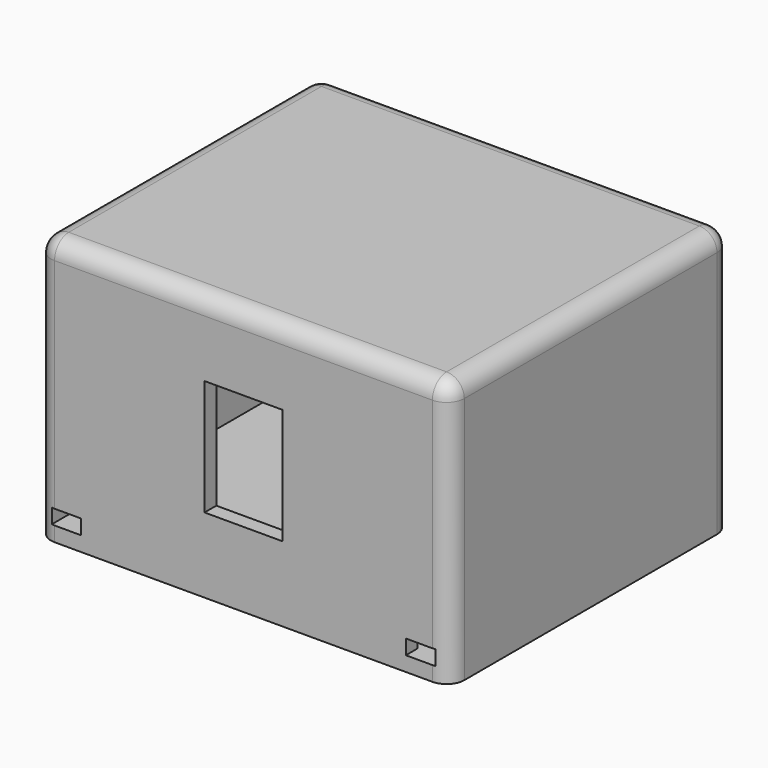
from build123d import *

# Parameters (mm, degrees)
F0_W         = 70
F0_H         = 45
F0_W_2       = 20.7
F0_H_2       = 27.2
F0_W_3       = 25.5
F0_H_3       = 32.8
F1_DEPTH     = 2
F2_W         = 70
F2_H         = 45
F2_W_2       = 65
F2_H_2       = 40
F3_DEPTH     = 55
F4_W         = 70
F4_H         = 45
F4_W_2       = 13.2
F4_H_2       = 19.6
F5_DEPTH     = 2.5
F6_W         = 5
F6_H         = 2.5
F7_DEPTH     = 59.501
F8_T1_DEPTH  = 64
F8_T3_DEPTH  = 49.5
F8_T5_DEPTH  = 53.5
F8_S9_W      = 3
F8_S9_H      = 3
F8_T10_DEPTH = 3
F8_S15_W     = 3
F8_S15_H     = 3
F8_T16_DEPTH = 3
F8_S21_W     = 3
F8_S21_H     = 3
F8_T22_DEPTH = 3
F8_S27_W     = 3
F8_S27_H     = 3
F8_T28_DEPTH = 3


# Not quite as in the source:
# - a fillet or chamfer that OpenCascade refuses, or shapes differently, is made with other operations: its cross-section is extruded or revolved along the edge and cut away or added


with BuildPart() as f1:
    # F0 (on Front) → F1 (new body)
    with BuildSketch(Plane.XZ):
        Rectangle(F0_W, F0_H)
        with Locations((17.65, -1.9)):
            Rectangle(F0_W_2, F0_H_2, mode=Mode.SUBTRACT)
        with Locations((-15.25, 0.9)):
            Rectangle(F0_W_3, F0_H_3, mode=Mode.SUBTRACT)
    extrude(amount=F1_DEPTH)

    # F2 (on face) → F3 (join)
    with BuildSketch(Plane.XZ.offset(2)):
        Rectangle(F2_W, F2_H)
        Rectangle(F2_W_2, F2_H_2, mode=Mode.SUBTRACT)
    extrude(amount=F3_DEPTH)

    # F4 (on face) → F5 (join)
    with BuildSketch(Plane.XZ.offset(57)):
        Rectangle(F4_W, F4_H)
        Rectangle(F4_W_2, F4_H_2, mode=Mode.SUBTRACT)
    extrude(amount=F5_DEPTH)

    # F6 (on face) → F7 (cut, through all)
    with BuildSketch(Plane(origin=(0, 0, 0), x_dir=(-1, 0, 0), z_dir=(0, 1, 0))):
        with Locations((-30, -18.75)):
            Rectangle(F6_W, F6_H)
        with Locations((30, -18.75)):
            Rectangle(F6_W, F6_H)
    extrude(amount=-F7_DEPTH, mode=Mode.SUBTRACT)

    # F8: fillet of radius 3 on 8 edges, made by hand

    # F8_s2 → F8_t1 (cut)
    with BuildSketch(Plane.YZ.offset(-32)):
        with BuildLine():
            ThreePointArc((-56.5, 22.5), (-58.6213203436, 21.6213203436), (-59.5, 19.5))
            Line((-59.5, 19.5), (-59.5, 22.5))
            Line((-59.5, 22.5), (-56.5, 22.5))
        make_face()
        with BuildLine():
            ThreePointArc((-3, 22.5), (-0.8786796564, 21.6213203436), (0, 19.5))
            Line((0, 19.5), (0, 22.5))
            Line((0, 22.5), (-3, 22.5))
        make_face()
    extrude(amount=F8_T1_DEPTH, mode=Mode.SUBTRACT)

    # F8_s4 → F8_t3 (cut)
    with BuildSketch(Plane.XY.offset(-30)):
        with BuildLine():
            ThreePointArc((32, -59.5), (34.1213203436, -58.6213203436), (35, -56.5))
            Line((35, -56.5), (35, -59.5))
            Line((35, -59.5), (32, -59.5))
        make_face()
        with BuildLine():
            ThreePointArc((-35, -56.5), (-34.1213203436, -58.6213203436), (-32, -59.5))
            Line((-32, -59.5), (-35, -59.5))
            Line((-35, -59.5), (-35, -56.5))
        make_face()
        with BuildLine():
            ThreePointArc((32, 0), (34.1213203436, -0.8786796564), (35, -3))
            Line((35, -3), (35, 0))
            Line((35, 0), (32, 0))
        make_face()
        with BuildLine():
            ThreePointArc((-32, 0), (-34.1213203436, -0.8786796564), (-35, -3))
            Line((-35, -3), (-35, 0))
            Line((-35, 0), (-32, 0))
        make_face()
    extrude(amount=F8_T3_DEPTH, mode=Mode.SUBTRACT)

    # F8_s6 → F8_t5 (cut)
    with BuildSketch(Plane.XZ.offset(3)):
        with BuildLine():
            ThreePointArc((32, 22.5), (34.1213203436, 21.6213203436), (35, 19.5))
            Line((35, 19.5), (35, 22.5))
            Line((35, 22.5), (32, 22.5))
        make_face()
        with BuildLine():
            ThreePointArc((-32, 22.5), (-34.1213203436, 21.6213203436), (-35, 19.5))
            Line((-35, 19.5), (-35, 22.5))
            Line((-35, 22.5), (-32, 22.5))
        make_face()
    extrude(amount=F8_T5_DEPTH, mode=Mode.SUBTRACT)


with BuildPart() as f8_tool8:
    # F8_s9 → F8_t10 (new body)
    with BuildSketch(Plane.XY.offset(19.5)):
        with Locations((33.5, -58)):
            Rectangle(F8_S9_W, F8_S9_H)
    extrude(amount=F8_T10_DEPTH)

    # F8_s11 → F8_t12 (revolve, cut)
    with BuildSketch(Plane(origin=(32, -56.5, 19.5), x_dir=(-0.7071067812, 0.7071067812, 0), z_dir=(0.7071067812, 0.7071067812, 0))):
        with BuildLine():
            ThreePointArc((0, -3), (3, 0), (0, 3))
            Line((0, 3), (0, -3))
        make_face()
    revolve(axis=Axis((32, -56.5, 19.5), (0, 0, 1)), mode=Mode.SUBTRACT)


with BuildPart() as f1_1:
    add(f1.part)

    # F8_t7: cut F8_tool8
    add(f8_tool8.part, mode=Mode.SUBTRACT)


with BuildPart() as f8_tool14:
    # F8_s15 → F8_t16 (new body)
    with BuildSketch(Plane.XY.offset(19.5)):
        with Locations((-33.5, -58)):
            Rectangle(F8_S15_W, F8_S15_H)
    extrude(amount=F8_T16_DEPTH)

    # F8_s17 → F8_t18 (revolve, cut)
    with BuildSketch(Plane(origin=(-32, -56.5, 19.5), x_dir=(0.7071067812, 0.7071067812, 0), z_dir=(0.7071067812, -0.7071067812, 0))):
        with BuildLine():
            ThreePointArc((0, -3), (3, 0), (0, 3))
            Line((0, 3), (0, -3))
        make_face()
    revolve(axis=Axis((-32, -56.5, 19.5), (0, 0, 1)), mode=Mode.SUBTRACT)


with BuildPart() as f1_2:
    add(f1_1.part)

    # F8_t13: cut F8_tool14
    add(f8_tool14.part, mode=Mode.SUBTRACT)


with BuildPart() as f8_tool20:
    # F8_s21 → F8_t22 (new body)
    with BuildSketch(Plane.XY.offset(19.5)):
        with Locations((33.5, -1.5)):
            Rectangle(F8_S21_W, F8_S21_H)
    extrude(amount=F8_T22_DEPTH)

    # F8_s23 → F8_t24 (revolve, cut)
    with BuildSketch(Plane(origin=(32, -3, 19.5), x_dir=(-0.7071067812, -0.7071067812, 0), z_dir=(-0.7071067812, 0.7071067812, 0))):
        with BuildLine():
            ThreePointArc((0, -3), (3, 0), (0, 3))
            Line((0, 3), (0, -3))
        make_face()
    revolve(axis=Axis((32, -3, 19.5), (0, 0, 1)), mode=Mode.SUBTRACT)


with BuildPart() as f1_3:
    add(f1_2.part)

    # F8_t19: cut F8_tool20
    add(f8_tool20.part, mode=Mode.SUBTRACT)


with BuildPart() as f8_tool26:
    # F8_s27 → F8_t28 (new body)
    with BuildSketch(Plane.XY.offset(19.5)):
        with Locations((-33.5, -1.5)):
            Rectangle(F8_S27_W, F8_S27_H)
    extrude(amount=F8_T28_DEPTH)

    # F8_s29 → F8_t30 (revolve, cut)
    with BuildSketch(Plane(origin=(-32, -3, 19.5), x_dir=(0.7071067812, -0.7071067812, 0), z_dir=(-0.7071067812, -0.7071067812, 0))):
        with BuildLine():
            ThreePointArc((0, -3), (3, 0), (0, 3))
            Line((0, 3), (0, -3))
        make_face()
    revolve(axis=Axis((-32, -3, 19.5), (0, 0, 1)), mode=Mode.SUBTRACT)


with BuildPart() as f1_4:
    add(f1_3.part)

    # F8_t25: cut F8_tool26
    add(f8_tool26.part, mode=Mode.SUBTRACT)


solid = f1_4.part
